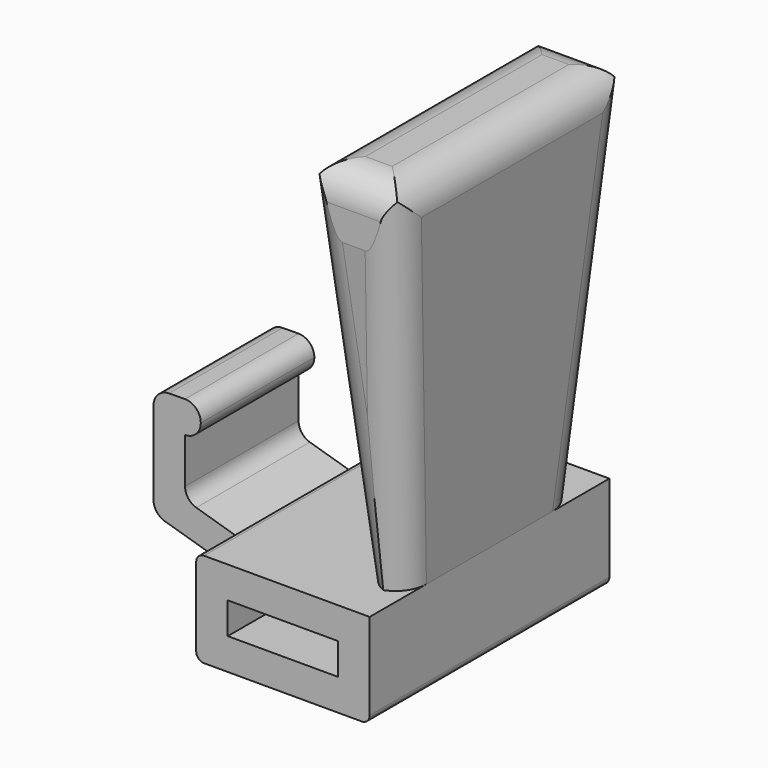
from build123d import *

# Parameters (mm, degrees)
F0_W         = 7
F0_H         = 2
F1_DEPTH     = 9.5
F2_DEPTH     = 9
F0_W_2       = 1
F3_DEPTH     = 4.5
F4_R         = 0.99999
F5_SIZE2     = 2
F5_SIZE      = 20
F5_2_SIZE2   = 2
F5_2_SIZE    = 20
F6_T1_DEPTH  = 49.9673321511
F6_T3_DEPTH  = 49.9117147518
F6_T5_DEPTH  = 49.9673321511
F6_T7_DEPTH  = 49.9117147518
F6_T9_DEPTH  = 28.6748999233
F6_T11_DEPTH = 28.841948309
F6_T13_DEPTH = 16
F7_R         = 0.5


# Not quite as in the source:
# - a fillet or chamfer that OpenCascade refuses, or shapes differently, is made with other operations: its cross-section is extruded or revolved along the edge and cut away or added
# - a fillet or chamfer is up to 0.001 mm smaller than in the source, because OpenCascade refuses the exact size


with BuildPart() as f1:
    # F0 (on Front) → F1 (new body, symmetric)
    with BuildSketch(Plane.XZ):
        Polygon((-30.0965141803, 12.928980055), (-19.0965141803, 12.928980055), (-19.0965141803, 18.928980055), (-30.0965141803, 18.928980055), (-30.0965141803, 16.928980055), (-30.0965141803, 14.928980055), align=None)
        with Locations((-24.5965141803, 15.928980055)):
            Rectangle(F0_W, F0_H, mode=Mode.SUBTRACT)
    extrude(amount=F1_DEPTH, both=True)

    # F0 (on Front) → F3 (join, symmetric)
    with BuildSketch(Plane.XZ):
        with Locations((-34.3048012789, 22.9472189589)):
            Rectangle(F0_W_2, F0_H)
        Polygon((-36.8047181128, 18.928980055), (-34.8048012789, 18.3327200564), (-34.8048012789, 21.9472189589), (-34.8048012789, 23.9472189589), (-36.8047181128, 23.928980055), align=None)
        Polygon((-36.8047181128, 16.928980055), (-30.0965141803, 14.928980055), (-30.0965141803, 16.928980055), (-34.8048012789, 18.3327200564), (-36.8047181128, 18.928980055), align=None)
    extrude(amount=F3_DEPTH, both=True)

    # F4 (radius 1 in the source; OpenCascade refuses exactly that, so slightly less here)
    f4_edges = [f1.edges().sort_by_distance(p)[0] for p in [
        (-36.804718, 0, 16.92898),
        (-36.804718, 0, 23.92898),
        (-33.804801, 0, 23.947219),
        (-33.804801, 0, 21.947219),
        (-34.804801, 0, 18.33272),
    ]]
    fillet(f4_edges, radius=F4_R)

    # F7
    f7_edges = [f1.edges().sort_by_distance(p)[0] for p in [
        (-30.096514, 0, 18.92898),
        (-30.096514, 0, 12.92898),
        (-19.096514, 0, 12.92898),
    ]]
    fillet(f7_edges, radius=F7_R)


with BuildPart() as f2:
    # F0 (on Front) → F2 (new body, symmetric)
    with BuildSketch(Plane.XZ):
        Polygon((-21.5954088979, 18.9560896729), (-19.0965141803, 18.928980055), (-17.531296789, 42.8778859699), (-23.531296789, 42.8778859699), align=None)
    extrude(amount=F2_DEPTH, both=True)

    # F5
    f5_edges = [f2.edges().sort_by_distance(p)[0] for p in [
        (-20.345962, -9, 18.942535),
    ]]
    f5_side = f2.faces().sort_by_distance((-20.450789, -9, 32.553702))[0]
    chamfer(f5_edges, length=F5_SIZE, length2=F5_SIZE2, reference=f5_side)

    # F5#2
    f5_2_edges = [f2.edges().sort_by_distance(p)[0] for p in [
        (-20.345962, 9, 18.942535),
    ]]
    f5_2_side = f2.faces().sort_by_distance((-20.450789, 9, 32.553702))[0]
    chamfer(f5_2_edges, length=F5_2_SIZE, length2=F5_2_SIZE2, reference=f5_2_side)

    # F6: fillet of radius 2 on 8 edges, made by hand

    # F6_s2 → F6_t1 (cut)
    with BuildSketch(Plane(origin=(4.1043145221, -6.2839672171, 62.7988437139), x_dir=(-0.8372400542, -0.5468355251, 0), z_dir=(-0.0648946801, 0.0993578929, -0.9929333762))):
        with BuildLine():
            ThreePointArc((18.7230377702, 8.4578509385), (19.9843267844, 7.5993584569), (21.4840038751, 7.8801215992))
            Line((21.4840038751, 7.8801215992), (19.8162152443, 6.7959541073))
            Line((19.8162152443, 6.7959541073), (18.7230377702, 8.4578509385))
        make_face()
    extrude(amount=F6_T1_DEPTH, mode=Mode.SUBTRACT)

    # F6_s4 → F6_t3 (cut)
    with BuildSketch(Plane(origin=(-5.3123669205, -6.5583508113, 65.6449993364), x_dir=(-0.7770579233, 0.6294290936, 0), z_dir=(0.0802650099, 0.099090688, -0.9918359561))):
        with BuildLine():
            ThreePointArc((10.8285170374, -15.2199185563), (12.2892990823, -15.648377047), (13.6285019913, -14.9245010705))
            Line((13.6285019913, -14.9245010705), (12.3748799347, -16.4595175875))
            Line((12.3748799347, -16.4595175875), (10.8285170374, -15.2199185563))
        make_face()
    extrude(amount=F6_T3_DEPTH, mode=Mode.SUBTRACT)

    # F6_s6 → F6_t5 (cut)
    with BuildSketch(Plane(origin=(4.1043145221, 6.2839672171, 62.7988437139), x_dir=(0.8372400542, -0.5468355251, 0), z_dir=(-0.0648946801, -0.0993578929, -0.9929333762))):
        with BuildLine():
            ThreePointArc((-18.7230377702, 8.4578509385), (-19.9843267844, 7.5993584569), (-21.4840038751, 7.8801215992))
            Line((-21.4840038751, 7.8801215992), (-19.8162152443, 6.7959541073))
            Line((-19.8162152443, 6.7959541073), (-18.7230377702, 8.4578509385))
        make_face()
    extrude(amount=F6_T5_DEPTH, mode=Mode.SUBTRACT)

    # F6_s8 → F6_t7 (cut)
    with BuildSketch(Plane(origin=(-5.3123669205, 6.5583508113, 65.6449993364), x_dir=(0.7770579233, 0.6294290936, 0), z_dir=(0.0802650099, -0.099090688, -0.9918359561))):
        with BuildLine():
            ThreePointArc((-10.8285170374, -15.2199185563), (-12.2892990823, -15.648377047), (-13.6285019913, -14.9245010705))
            Line((-13.6285019913, -14.9245010705), (-12.3748799347, -16.4595175875))
            Line((-12.3748799347, -16.4595175875), (-10.8285170374, -15.2199185563))
        make_face()
    extrude(amount=F6_T7_DEPTH, mode=Mode.SUBTRACT)

    # F6_s10 → F6_t9 (cut)
    with BuildSketch(Plane.XZ.offset(-14.3374499616)):
        with BuildLine():
            ThreePointArc((-17.6705346141, 40.7474511872), (-18.2066758753, 42.2452064215), (-19.6662767737, 42.8778859699))
            Line((-19.6662767737, 42.8778859699), (-17.531296789, 42.8778859699))
            Line((-17.531296789, 42.8778859699), (-17.6705346141, 40.7474511872))
        make_face()
    extrude(amount=F6_T9_DEPTH, mode=Mode.SUBTRACT)

    # F6_s12 → F6_t11 (cut)
    with BuildSketch(Plane.XZ.offset(-14.4209741545)):
        with BuildLine():
            ThreePointArc((-21.3629071272, 42.8778859699), (-22.8330513347, 42.2338638491), (-23.3563901519, 40.7165619789))
            Line((-23.3563901519, 40.7165619789), (-23.531296789, 42.8778859699))
            Line((-23.531296789, 42.8778859699), (-21.3629071272, 42.8778859699))
        make_face()
    extrude(amount=F6_T11_DEPTH, mode=Mode.SUBTRACT)

    # F6_s14 → F6_t13 (cut)
    with BuildSketch(Plane.YZ.offset(-28.531296789)):
        with BuildLine():
            ThreePointArc((-9, 40.8778859699), (-8.4142135624, 42.2920995322), (-7, 42.8778859699))
            Line((-7, 42.8778859699), (-9, 42.8778859699))
            Line((-9, 42.8778859699), (-9, 40.8778859699))
        make_face()
        with BuildLine():
            ThreePointArc((9, 40.8778859699), (8.4142135624, 42.2920995322), (7, 42.8778859699))
            Line((7, 42.8778859699), (9, 42.8778859699))
            Line((9, 42.8778859699), (9, 40.8778859699))
        make_face()
    extrude(amount=F6_T13_DEPTH, mode=Mode.SUBTRACT)


solid = Compound([f1.part, f2.part])
